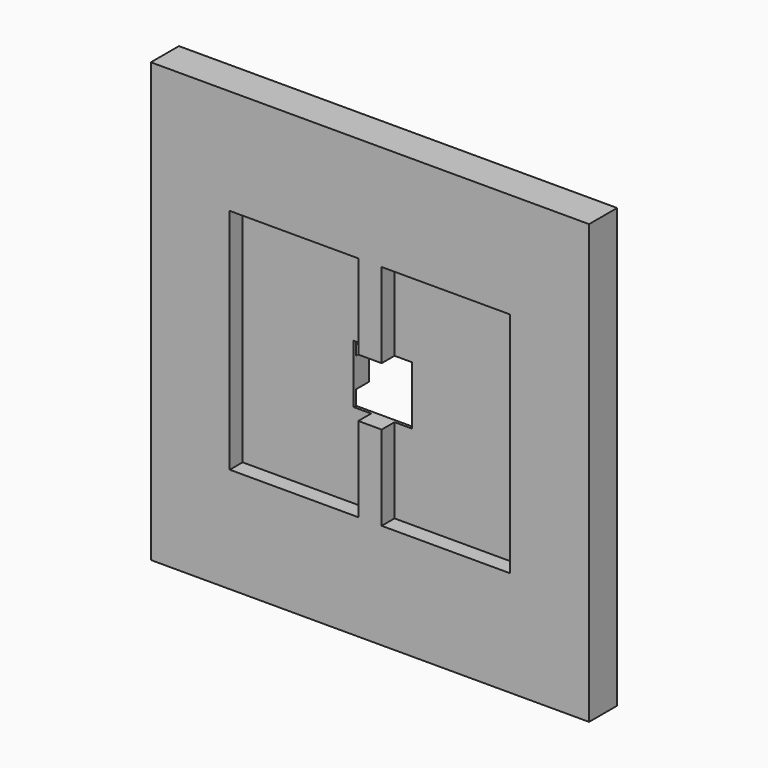
from build123d import *

# Parameters (mm, degrees)
F0_W     = 75
F0_H     = 75
F0_W_2   = 10
F0_H_2   = 10
F1_DEPTH = 6
F3_DEPTH = 2.75
F5_DEPTH = 2.75


# Not quite as in the source:
# - a feature names something its author has since deleted; it is built from what else it names


with BuildPart() as f1:
    # F0 (on Front) → F1 (new body)
    with BuildSketch(Plane.XZ):
        Rectangle(F0_W, F0_H)
        Rectangle(F0_W_2, F0_H_2, mode=Mode.SUBTRACT)
    extrude(amount=F1_DEPTH)

    # F2 (on face) → F3 (cut)
    with BuildSketch(Plane.XZ.offset(6)):
        Polygon((-24, -19.5), (-2, -19.5), (-2, -5), (-5, -5), (-5, 5), (-2, 5), (-2, 19.5), (-24, 19.5), align=None)
        Polygon((2, -19.5), (24, -19.5), (24, 19.5), (2, 19.5), (2, 5), (5, 5), (5, -5), (2, -5), align=None)
    extrude(amount=-F3_DEPTH, mode=Mode.SUBTRACT)

    # F4 (on face) → F5 (cut)
    with BuildSketch(Plane(origin=(0, 0, 0), x_dir=(-1, 0, 0), z_dir=(0, 1, 0))):
        Polygon((-19.5, -24), (19.5, -24), (19.5, -2.5302600116), (5, -2.5302600116), (5, -5), (-5, -5), (-5, -2.5302600116), (-19.5, -2.5302600116), align=None)
        Polygon((5, 2.5302600116), (19.5, 2.5302600116), (19.5, 24), (-19.5, 24), (-19.5, 2.5302600116), (-5, 2.5302600116), (-5, 5), (5, 5), align=None)
    extrude(amount=-F5_DEPTH, mode=Mode.SUBTRACT)


solid = f1.part
